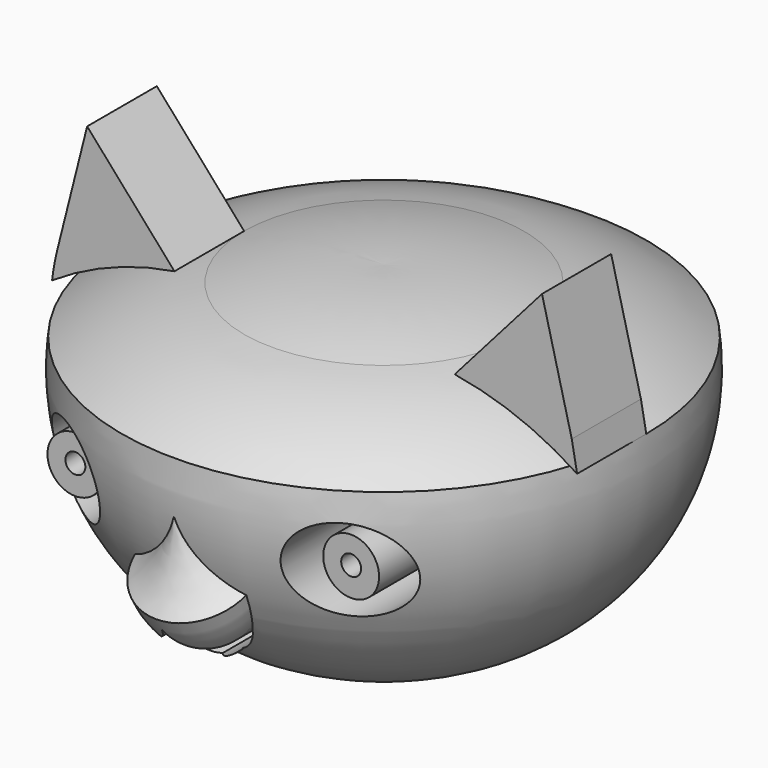
from build123d import *

# Parameters (mm, degrees)
F2_DEPTH      = 24.85668
F3_DEPTH      = 25.04527
F4_R          = 13.1489437665
F5_DEPTH      = 75.8785949149
F5_DEPTH_BACK = 25.4
F8_R          = 8.0324492067
F9_DEPTH      = 61.36749
F10_R         = 2.8666326471
F11_DEPTH     = 76.2
F14_DEPTH     = 25.4
F15_DEPTH     = 81.8650590714


# Not quite as in the source:
# - the program builds the solid bodies; features that only make, move or delete a surface that nothing else refers to are left out


with BuildPart() as f1:
    # F0 (on Front) → F1 (revolve)
    with BuildSketch(Plane.XZ):
        with BuildLine():
            Line((0, -64.6070092916), (0, 26.6700014472))
            ThreePointArc((0, 26.6700014472), (-20.2839717245, 25.9259113763), (-40.2189306915, 22.1061483026))
            ThreePointArc((-40.2189306915, 22.1061483026), (-58.5524469647, 17.1204069046), (-75.414945718, 8.3664608215))
            ThreePointArc((-75.414945718, 8.3664608215), (-55.793548621, -46.8114563829), (0, -64.6070092916))
        make_face()
    revolve(axis=Axis((0, 0, -18.9685039222), (0, 0, -1)))

    # F4 (on Front) → F5 (cut, two sides)
    with BuildSketch(Plane.XZ) as f5_sk:
        with Locations((-39.3632091582, -12.6932086423)):
            Circle(F4_R)
        with Locations((39.3632091582, -12.6932086423)):
            Circle(F4_R)
    extrude(amount=F5_DEPTH, mode=Mode.SUBTRACT)
    extrude(f5_sk.sketch, amount=-F5_DEPTH_BACK, mode=Mode.SUBTRACT)

    # F6 (on Right) → F7 (revolve)
    with BuildSketch(Plane.YZ):
        with BuildLine():
            ThreePointArc((-75.5887702107, -6.4179147594), (-76.967885123, -18.5845814047), (-81.8640589714, -29.8076476902))
            ThreePointArc((-81.8640589714, -29.8076476902), (-70.4255242509, -42.7414452162), (-54.1957207024, -48.633530736))
            Line((-54.1957207024, -48.633530736), (-75.5887702107, -6.4179147594))
        make_face()
    revolve(axis=Axis((0, -64.8922454566, -27.5257227477), (0, 0.4520287519, -0.8920033674)))

    # F13 (on Front) → F14 (cut)
    with BuildSketch(Plane.XZ):
        with BuildLine():
            ThreePointArc((0, -33.230535686), (-6.4422735782, -38.6430436558), (-13.6915519834, -34.3714989722))
            ThreePointArc((-13.6915519834, -34.3714989722), (-8.4358947574, -42.8073922995), (0, -48.0630472302))
            ThreePointArc((0, -48.0630472302), (8.4358947574, -42.8073922995), (13.6915519834, -34.3714989722))
            ThreePointArc((13.6915519834, -34.3714989722), (6.4422735782, -38.6430436558), (0, -33.230535686))
        make_face()
    extrude(amount=F14_DEPTH, mode=Mode.SUBTRACT)

    # F13 (on Front) → F15 (cut, through all)
    with BuildSketch(Plane.XZ):
        with BuildLine():
            ThreePointArc((0, -33.230535686), (-6.4422735782, -38.6430436558), (-13.6915519834, -34.3714989722))
            ThreePointArc((-13.6915519834, -34.3714989722), (-8.4358947574, -42.8073922995), (0, -48.0630472302))
            ThreePointArc((0, -48.0630472302), (8.4358947574, -42.8073922995), (13.6915519834, -34.3714989722))
            ThreePointArc((13.6915519834, -34.3714989722), (6.4422735782, -38.6430436558), (0, -33.230535686))
        make_face()
    extrude(amount=F15_DEPTH, mode=Mode.SUBTRACT)


with BuildPart() as f2:
    # F0 (on Front) → F2 (new body)
    with BuildSketch(Plane.XZ):
        with BuildLine():
            Line((65.3201043606, 50.6302118301), (40.2189306915, 22.1061483026))
            ThreePointArc((40.2189306915, 22.1061483026), (58.5524469647, 17.1204069046), (75.414945718, 8.3664608215))
            Line((75.414945718, 8.3664608215), (73.8773271441, 16.6865773499))
            Line((73.8773271441, 16.6865773499), (65.3201043606, 50.6302118301))
        make_face()
    extrude(amount=F2_DEPTH)


with BuildPart() as f3:
    # F0 (on Front) → F3 (new body)
    with BuildSketch(Plane.XZ):
        with BuildLine():
            ThreePointArc((-75.414945718, 8.3664608215), (-58.5524469647, 17.1204069046), (-40.2189306915, 22.1061483026))
            Line((-40.2189306915, 22.1061483026), (-65.3201043606, 50.6302118301))
            Line((-65.3201043606, 50.6302118301), (-73.8773271441, 16.6865773499))
            ThreePointArc((-73.8773271441, 16.6865773499), (-74.7797401426, 12.5512100318), (-75.414945718, 8.3664608215))
        make_face()
    extrude(amount=F3_DEPTH)


with BuildPart() as f9:
    # F8 (on Front) → F9 (new body)
    with BuildSketch(Plane.XZ):
        with Locations((-39.648450911, -11.8374861777)):
            Circle(F8_R)
    extrude(amount=F9_DEPTH)


with BuildPart() as f9b:
    # F8 (on Front) → F9, piece 2 (new body)
    with BuildSketch(Plane.XZ):
        with Locations((39.648450911, -11.8374861777)):
            Circle(F8_R)
    extrude(amount=F9_DEPTH)


with BuildPart() as f11_tool:
    # F10 (on Front) → F11 (new body)
    with BuildSketch(Plane.XZ):
        with Locations((-39.648450911, -11.5522462875)):
            Circle(F10_R)
        with Locations((39.648450911, -11.5522462875)):
            Circle(F10_R)
    extrude(amount=F11_DEPTH)


with BuildPart() as f9_1:
    add(f9.part)

    # F11: cut by f11_tool
    add(f11_tool.part, mode=Mode.SUBTRACT)


with BuildPart() as f9b_1:
    add(f9b.part)

    # F11: cut by f11_tool
    add(f11_tool.part, mode=Mode.SUBTRACT)


solid = Compound([f1.part, f2.part, f3.part, f9_1.part, f9b_1.part])
